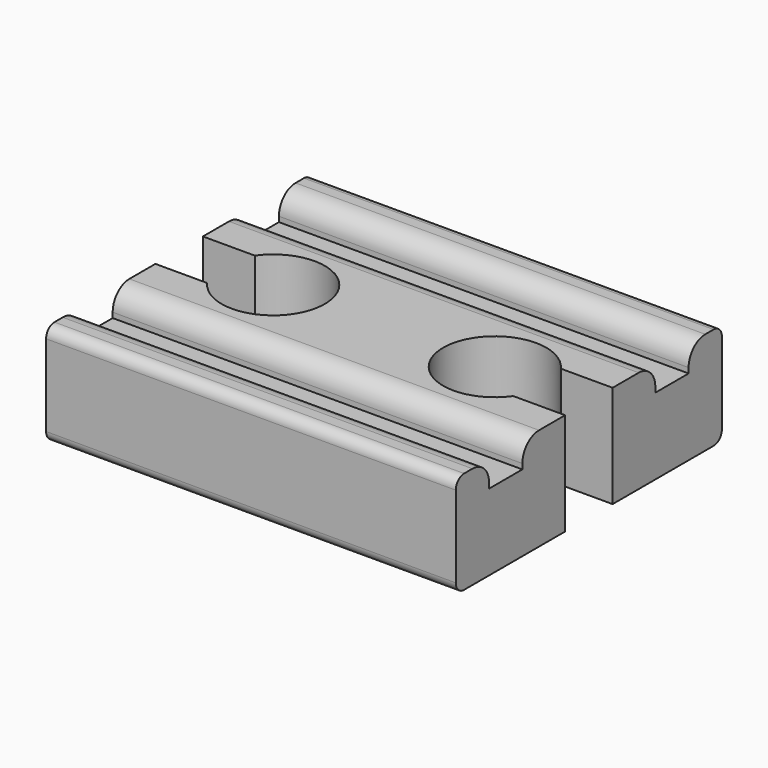
from build123d import *

# Parameters (mm, degrees)
F0_W     = 50
F0_H     = 40.6
F1_DEPTH = 12.5
F3_DEPTH = 12.501
F4_W     = 50
F4_H     = 5.08
F5_DEPTH = 3.175
F6_R     = 1.27
F7_R     = 2.54


# Not quite as in the source:
# - a pattern or mirror of a feature is missing from the dataset's text; its kind, count and spacing are read off the source's solid


with BuildPart() as f1:
    # F0 (on Top) → F1 (new body)
    with BuildSketch(Plane.XY):
        Rectangle(F0_W, F0_H)
    extrude(amount=F1_DEPTH)

    # F2 (on Top) → F3 (cut, through all)
    with BuildSketch(Plane.XY):
        with BuildLine():
            Line((25, -2.794), (25, 3.625))
            Line((25, 3.625), (18.6726085627, 3.625))
            ThreePointArc((18.6726085627, 3.625), (7.22, 0), (18.6726085627, -3.625))
            Line((18.6726085627, -3.625), (25, -3.625))
            Line((25, -3.625), (25, -2.794))
        make_face()
    f3 = extrude(amount=F3_DEPTH, mode=Mode.SUBTRACT)

    # F3_copies: F3 across plane
    add(f3.mirror(Plane(origin=(0, 0, 0), x_dir=(0, 0, -1), z_dir=(-1, 0, 0))), mode=Mode.SUBTRACT)

    # F4 (on face) → F5 (cut)
    with BuildSketch(Plane.XY.offset(12.5)):
        with Locations((0, 12.68)):
            Rectangle(F4_W, F4_H)
    f5 = extrude(amount=-F5_DEPTH, mode=Mode.SUBTRACT)

    # F5_copies: F5 across plane
    add(f5.mirror(Plane(origin=(0, 0, 0), x_dir=(0, 0, -1), z_dir=(0, -1, 0))), mode=Mode.SUBTRACT)

    # F6
    f6_edges = [f1.edges().sort_by_distance(p)[0] for p in [
        (0, 20.3, 12.5),
        (0, -20.3, 12.5),
        (0, 20.3, 0),
        (0, -20.3, 0),
    ]]
    fillet(f6_edges, radius=F6_R)

    # F7
    f7_edges = [f1.edges().sort_by_distance(p)[0] for p in [
        (0, 15.22, 12.5),
        (0, 10.14, 12.5),
        (0, -10.14, 12.5),
        (0, -15.22, 12.5),
    ]]
    fillet(f7_edges, radius=F7_R)


solid = f1.part
